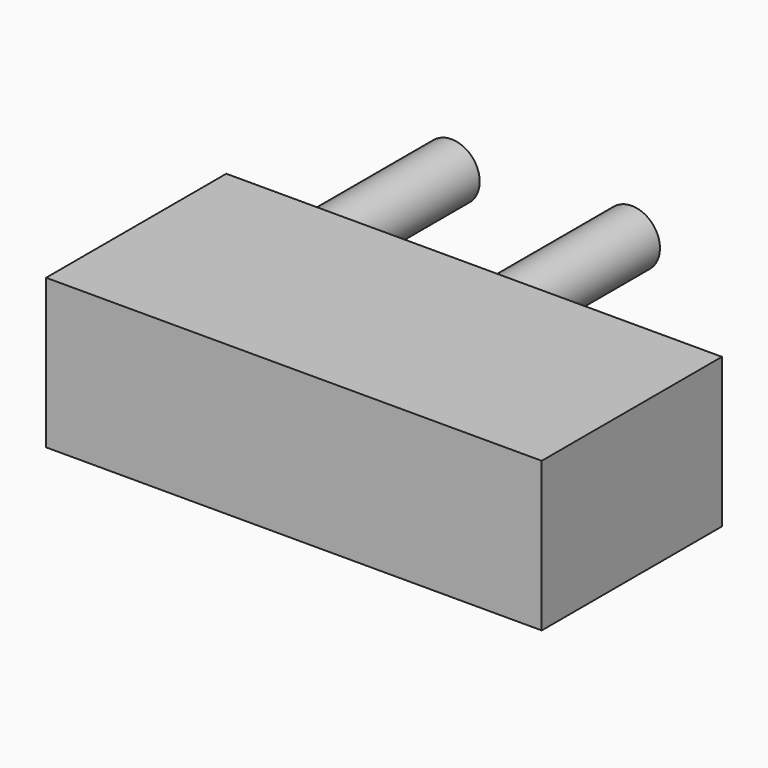
from build123d import *

# Parameters (mm, degrees)
F0_W     = 30.4900507075
F0_H     = 16.8403594638
F0_R     = 3.175
F1_DEPTH = 25.4
F2_R     = 3.175
F3_DEPTH = 25.4
F4_DEPTH = 25.4


# Not quite as in the source:
# - a feature names something its author has since deleted; it is built from what else it names


with BuildPart() as f1:
    # F0 (on Front) → F1 (new body)
    with BuildSketch(Plane.XZ):
        Rectangle(F0_W, F0_H)
        with Locations((-7.6225126769, 0)):
            Circle(F0_R, mode=Mode.SUBTRACT)
        with Locations((7.6225126769, 0)):
            Circle(F0_R, mode=Mode.SUBTRACT)
        with Locations((-7.6225126769, 0)):
            Circle(F0_R)
        with Locations((7.6225126769, 0)):
            Circle(F0_R)
    extrude(amount=F1_DEPTH)

    # F2 (on face) → F3 (join)
    with BuildSketch(Plane(origin=(0, 0, 0), x_dir=(-1, 0, 0), z_dir=(0, 1, 0))):
        with Locations((10.1633502358, 0)):
            Circle(F2_R)
        with Locations((-10.1633502358, 0)):
            Circle(F2_R)
    extrude(amount=F3_DEPTH)

    # F4 (add): a face of the model
    f4_faces = [f1.faces().sort_by_distance(p)[0] for p in [
        (15.2450253537, -12.7, 0),
    ]]
    extrude(f4_faces, amount=F4_DEPTH)


solid = f1.part
